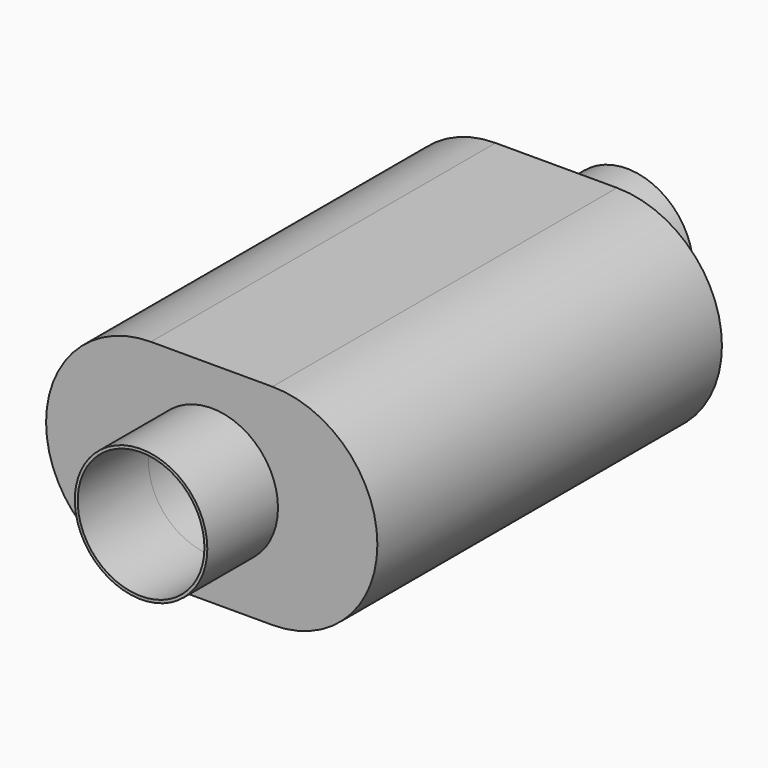
from build123d import *
from build123d import SkipClean  # not in build123d's __all__

# Parameters (mm, degrees)
F1_DEPTH = 247.65
F2_R     = 38.1
F2_R_2   = 36.449
F3_DEPTH = 50.8
F4_R     = 38.1
F4_R_2   = 36.449
F5_DEPTH = 50.8
F6_DEPTH = 330.2


with BuildPart() as f1:
    # F0 (on Front) → F1 (new body)
    with BuildSketch(Plane.XZ):
        with BuildLine():
            Line((34.925, 60.325), (-34.925, 60.325))
            ThreePointArc((-34.925, 60.325), (-95.25, 0), (-34.925, -60.325))
            Line((-34.925, -60.325), (34.925, -60.325))
            ThreePointArc((34.925, -60.325), (95.25, 0), (34.925, 60.325))
        make_face()
    extrude(amount=F1_DEPTH)

    # F2 (on face) → F3 (join)
    with BuildSketch(Plane.XZ.offset(247.65)):
        Circle(F2_R)
        Circle(F2_R_2, mode=Mode.SUBTRACT)
    extrude(amount=F3_DEPTH)

    # F4 (on face) → F5 (join)
    with BuildSketch(Plane(origin=(0, 0, 0), x_dir=(-1, 0, 0), z_dir=(0, 1, 0))):
        Circle(F4_R)
        Circle(F4_R_2, mode=Mode.SUBTRACT)
    extrude(amount=F5_DEPTH)

    # F6 (cut): a face of the model
    f6_faces = [f1.faces().sort_by_distance(p)[0] for p in [
        (0, -247.65, 0),
    ]]
    with SkipClean():  # cleaning this boolean's faces spoils the solid; the shape is the same uncleaned
        extrude(f6_faces, amount=-F6_DEPTH, mode=Mode.SUBTRACT)


solid = f1.part
